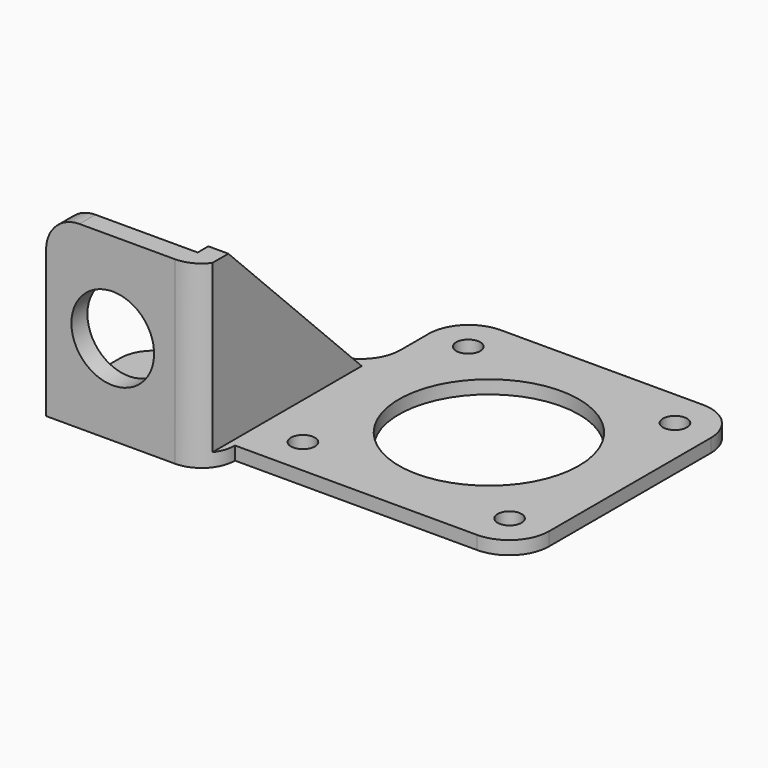
from build123d import *

# Parameters (mm, degrees)
F0_R         = 1.8
F0_R_2       = 13.5
F0_W         = 24.3372796029
F0_H         = 5
F1_DEPTH     = 2
F2_W         = 3
F2_H         = 30
F3_DEPTH     = 27
F4_W         = 20.3372796029
F4_H         = 3
F5_DEPTH     = 25
F7_SIZE      = 25
F8_SIZE      = 14
F9_R         = 4.99999
F10_T1_DEPTH = 2
F10_T3_DEPTH = 32
F6_R         = 6.2
F11_DEPTH    = 25


# Not quite as in the source:
# - a fillet or chamfer that OpenCascade refuses, or shapes differently, is made with other operations: its cross-section is extruded or revolved along the edge and cut away or added
# - a fillet or chamfer is up to 0.001 mm smaller than in the source, because OpenCascade refuses the exact size


with BuildPart() as f1:
    # F0 (on Top) → F1 (new body)
    with BuildSketch(Plane.XY):
        Polygon((21.15, -21.15), (21.15, 21.15), (-21.15, 21.15), (-21.15, 3.85), (-21.15, -21.15), align=None)
        with Locations((-15.5, -15.5)):
            Circle(F0_R, mode=Mode.SUBTRACT)
        with Locations((15.5, -15.5)):
            Circle(F0_R, mode=Mode.SUBTRACT)
        with Locations((-15.5, 15.5)):
            Circle(F0_R, mode=Mode.SUBTRACT)
        Circle(F0_R_2, mode=Mode.SUBTRACT)
        with Locations((15.5, 15.5)):
            Circle(F0_R, mode=Mode.SUBTRACT)
        Polygon((-21.15, -21.15), (-21.15, 3.85), (-45.5, 3.85), (-45.5, -21.15), (-21.1627203971, -21.15), align=None)
        with Locations((-33.3313601986, -23.65)):
            Rectangle(F0_W, F0_H)
    extrude(amount=F1_DEPTH)

    # F2 (on Top) → F3 (join)
    with BuildSketch(Plane.XY):
        with Locations((-23.6627203971, -11.15)):
            Rectangle(F2_W, F2_H)
    extrude(amount=F3_DEPTH)

    # F4 (on face) → F5 (join)
    with BuildSketch(Plane.XY.offset(2)):
        with Locations((-35.3313601986, -24.65)):
            Rectangle(F4_W, F4_H)
    extrude(amount=F5_DEPTH)

    # F7
    f7_edges = [f1.edges().sort_by_distance(p)[0] for p in [
        (-23.66272, 3.85, 27),
    ]]
    chamfer(f7_edges, length=F7_SIZE)

    # F8
    f8_edges = [f1.edges().sort_by_distance(p)[0] for p in [
        (-45.5, 3.85, 1),
    ]]
    chamfer(f8_edges, length=F8_SIZE)

    # F9 (radius 5 in the source; OpenCascade refuses exactly that, so slightly less here)
    f9_edges = [f1.edges().sort_by_distance(p)[0] for p in [
        (-45.5, -10.15, 1),
        (-31.5, 3.85, 1),
        (-21.16272, -26.15, 1),
        (-45.5, -24.65, 27),
    ]]
    fillet(f9_edges, radius=F9_R)

    # F10: fillet of radius 6 on 4 edges, made by hand

    # F10_s2 → F10_t1 (join)
    with BuildSketch(Plane.XY):
        with BuildLine():
            ThreePointArc((-27.15, 3.85), (-22.9073593129, 5.6073593129), (-21.15, 9.85))
            Line((-21.15, 9.85), (-21.15, 3.85))
            Line((-21.15, 3.85), (-27.15, 3.85))
        make_face()
    extrude(amount=F10_T1_DEPTH)

    # F10_s4 → F10_t3 (cut)
    with BuildSketch(Plane.XY.offset(-15)):
        with BuildLine():
            ThreePointArc((21.15, -15.15), (19.3926406871, -19.3926406871), (15.15, -21.15))
            Line((15.15, -21.15), (21.15, -21.15))
            Line((21.15, -21.15), (21.15, -15.15))
        make_face()
        with BuildLine():
            ThreePointArc((15.15, 21.15), (19.3926406871, 19.3926406871), (21.15, 15.15))
            Line((21.15, 15.15), (21.15, 21.15))
            Line((21.15, 21.15), (15.15, 21.15))
        make_face()
        with BuildLine():
            ThreePointArc((-21.15, 15.15), (-19.3926406871, 19.3926406871), (-15.15, 21.15))
            Line((-15.15, 21.15), (-21.15, 21.15))
            Line((-21.15, 21.15), (-21.15, 15.15))
        make_face()
    extrude(amount=F10_T3_DEPTH, mode=Mode.SUBTRACT)

    # F6 (on face) + F5_face1 (on face) → F11 (cut)
    with BuildSketch(Plane(origin=(0, -23.15, 0), x_dir=(-1, 0, 0), z_dir=(0, 1, 0))):
        with Locations((35.5, 13.5)):
            Circle(F6_R)
    with BuildSketch(Plane(origin=(-35.7425668405, -26.15, 13.3714329468), x_dir=(1, 0, 0), z_dir=(0, -1, 0))):
        with BuildLine():
            Line((-9.7574331595, -13.3714329468), (9.5798564434, -13.3714329468))
            Line((9.5798564434, -13.3714329468), (9.5798564434, 13.6285670532))
            Line((9.5798564434, 13.6285670532), (-4.7574431595, 13.6285670532))
            ThreePointArc((-4.7574431595, 13.6285670532), (-8.2929699944, 12.1641038881), (-9.7574331595, 8.6285770532))
            Line((-9.7574331595, 8.6285770532), (-9.7574331595, -13.3714329468))
        make_face()
    extrude(amount=-F11_DEPTH, dir=(0, 1, 0), mode=Mode.SUBTRACT)


solid = f1.part
